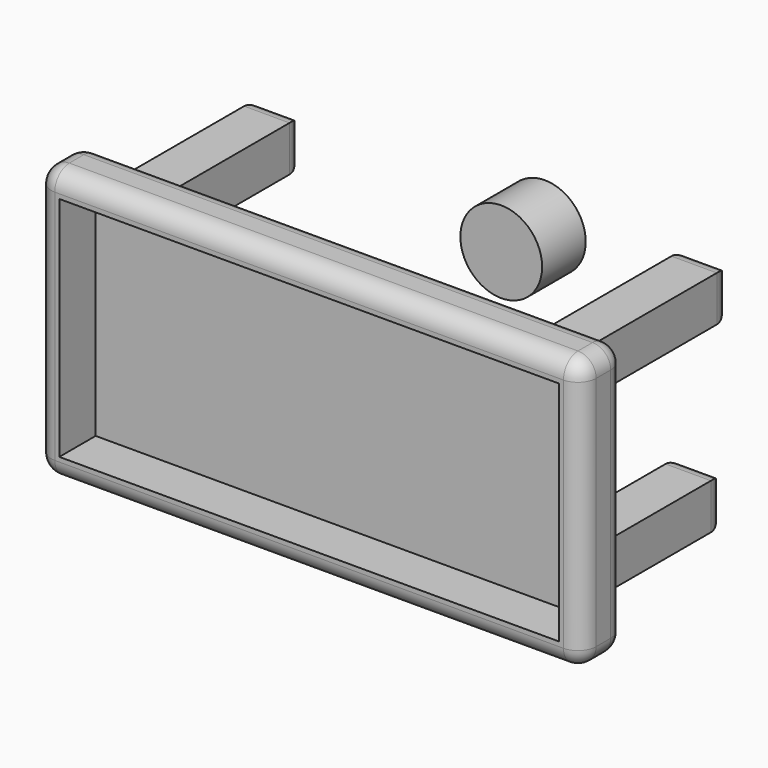
from build123d import *

# Parameters (mm, degrees)
F0_W     = 152.4
F0_H     = 76.2
F0_W_2   = 139.7
F0_H_2   = 63.5
F1_DEPTH = 15.24
F0_R     = 11.43
F2_DEPTH = 2.54
F3_R     = 5.08
F4_W     = 12.7
F4_H     = 12.7
F5_DEPTH = 49.53
F6_R     = 5.08


# Not quite as in the source:
# - a feature names something its author has since deleted; it is built from what else it names


with BuildPart() as f1:
    # F0 (on Front) → F1 (new body)
    with BuildSketch(Plane.XZ):
        with Locations((0, 2.523175699)):
            Rectangle(F0_W, F0_H)
        with Locations((0, 2.523175699)):
            Rectangle(F0_W_2, F0_H_2, mode=Mode.SUBTRACT)
    extrude(amount=F1_DEPTH)

    # F0 (on Front) → F2 (join)
    with BuildSketch(Plane.XZ):
        with Locations((0, 2.523175699)):
            Rectangle(F0_W_2, F0_H_2)
    extrude(amount=F2_DEPTH)

    # F3
    f3_edges = [f1.edges().sort_by_distance(p)[0] for p in [
        (-76.2, -15.24, 2.523176),
        (76.2, -15.24, 2.523176),
        (-76.2, -7.62, -35.576824),
        (76.2, -7.62, -35.576824),
        (0, 0, -35.576824),
        (0, -15.24, -35.576824),
        (76.2, -7.62, 40.623176),
        (76.2, 0, 2.523176),
        (-76.2, -7.62, 40.623176),
        (-76.2, 0, 2.523176),
        (0, 0, 40.623176),
        (0, -15.24, 40.623176),
    ]]
    fillet(f3_edges, radius=F3_R)

    # F4 (on Front) → F5 (join)
    with BuildSketch(Plane.XZ):
        with Locations((59.9117761264, 29.707653685)):
            Rectangle(F4_W, F4_H)
        with Locations((58.2590709269, -21.9867194656)):
            Rectangle(F4_W, F4_H)
        with Locations((-59.6288775811, -21.9100740052)):
            Rectangle(F4_W, F4_H)
        with Locations((-59.5799170583, 27.7787972095)):
            Rectangle(F4_W, F4_H)
    extrude(amount=-F5_DEPTH)

    # F6
    f6_edges = [f1.edges().sort_by_distance(p)[0] for p in [
        (58.259071, 49.53, -15.636719),
        (51.909071, 49.53, -21.986719),
        (58.259071, 49.53, -28.336719),
        (64.609071, 49.53, -21.986719),
        (-65.978878, 49.53, -21.910074),
        (-59.628878, 49.53, -28.260074),
        (-53.278878, 49.53, -21.910074),
        (-59.628878, 49.53, -15.560074),
        (66.261776, 49.53, 29.707654),
        (59.911776, 49.53, 36.057654),
        (53.561776, 49.53, 29.707654),
        (59.911776, 49.53, 23.357654),
        (-59.579917, 49.53, 34.128797),
        (-65.929917, 49.53, 27.778797),
        (-59.579917, 49.53, 21.428797),
        (-53.229917, 49.53, 27.778797),
    ]]
    fillet(f6_edges, radius=F6_R)


with BuildPart() as f1b:
    # F0 (on Front) → F1, piece 2 (new body)
    with BuildSketch(Plane.XZ):
        with Locations((53.7286363542, 61.4593066275)):
            Circle(F0_R)
    extrude(amount=F1_DEPTH)


solid = Compound([f1.part, f1b.part])
